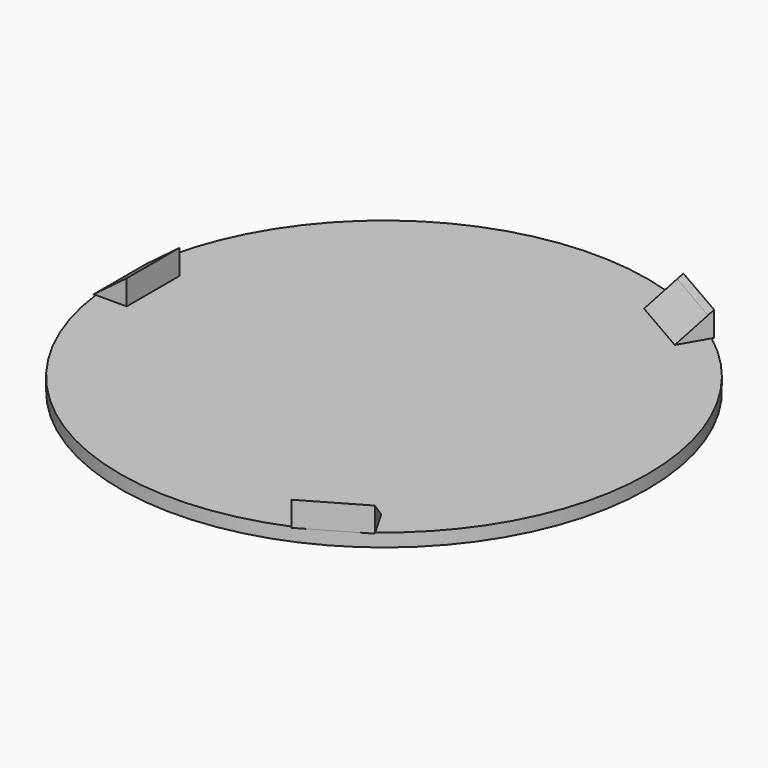
from build123d import *

# Parameters (mm, degrees)
F0_R     = 50.8
F1_DEPTH = 2.54
F3_DEPTH = 12.7
F5_DEPTH = 25.4
F7_DEPTH = 25.4
F9_DEPTH = 25.4


# Not quite as in the source:
# - a feature names something its author has since deleted; it is built from what else it names


with BuildPart() as f1:
    # F0 (on Top) → F1 (new body)
    with BuildSketch(Plane.XY):
        Circle(F0_R)
    extrude(amount=F1_DEPTH)

    # F2 (on face) → F3 (join)
    with BuildSketch(Plane.XY.offset(2.54)):
        Polygon((-50.8, 6.35), (-50.8, 0), (-50.8, -6.35), (-44.45, -6.35), (-44.45, 6.35), align=None)
        Polygon((16.725738686, -41.6698291982), (19.900738686, -47.1690905122), (30.899261314, -40.8190905122), (27.724261314, -35.3198291982), align=None)
        Polygon((27.724261314, 35.3198291982), (30.899261314, 40.8190905122), (19.900738686, 47.1690905122), (16.725738686, 41.6698291982), align=None)
    extrude(amount=F3_DEPTH)

    # F4 (on face) → F5 (cut)
    with BuildSketch(Plane.XZ.offset(6.35)):
        Polygon((-50.8, 15.24), (-50.8, 2.54), (-46.2367217033, 5.962595906), (-44.45, 7.3026908967), (-44.45, 15.24), align=None)
    extrude(amount=-F5_DEPTH, mode=Mode.SUBTRACT)

    # F6 (on face) → F7 (cut)
    with BuildSketch(Plane(origin=(5.499261314, 3.175, 0), x_dir=(-0.5, 0.8660254038, 0), z_dir=(0.8660254038, 0.5, 0))):
        Polygon((-50.0320994455, 6.7267423959), (-44.45, 2.54), (-44.45, 15.24), (-50.8, 15.24), (-50.8, 7.3026908967), align=None)
    extrude(amount=-F7_DEPTH, mode=Mode.SUBTRACT)

    # F8 (on face) → F9 (cut)
    with BuildSketch(Plane(origin=(-5.499261314, 3.175, 0), x_dir=(-0.5, -0.8660254038, 0), z_dir=(-0.8660254038, 0.5, 0))):
        Polygon((-50.8, 15.24), (-50.8, 7.3026908967), (-49.8044750842, 6.556017282), (-44.45, 2.54), (-44.45, 15.24), align=None)
    extrude(amount=-F9_DEPTH, mode=Mode.SUBTRACT)


solid = f1.part
